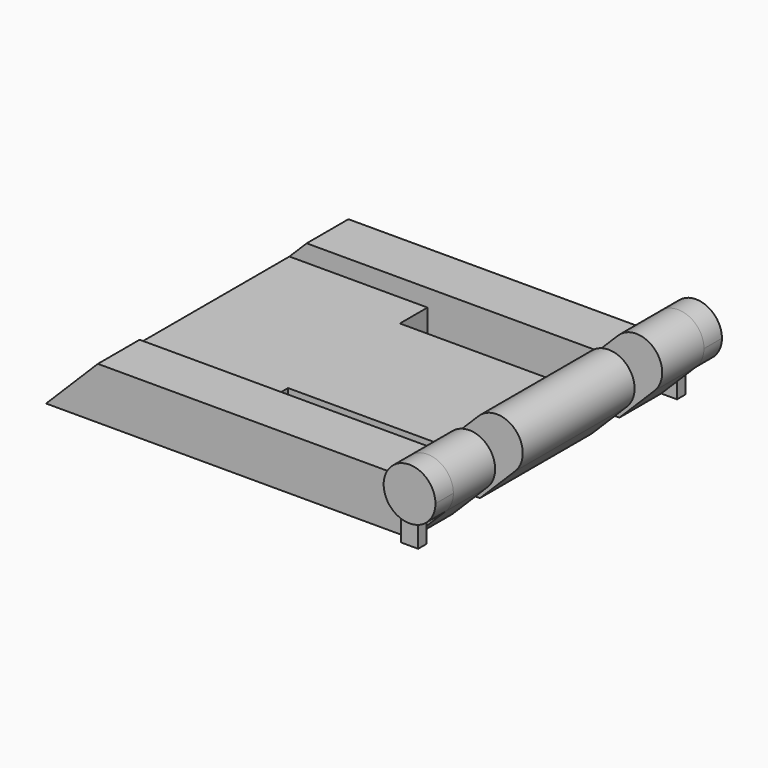
from build123d import *

# Parameters (mm, degrees)
F1_DEPTH  = 9.075
F3_DEPTH  = 1.3
F6_DEPTH  = 6.05
F7_W      = 15
F7_H      = 2
F8_DEPTH  = 4.601
F9_W      = 1
F9_H      = 0.6
F10_DEPTH = 3


with BuildPart() as f1:
    # F0 (on Front) → F1 (new body, symmetric)
    with BuildSketch(Plane.XZ):
        with BuildLine():
            Line((-3.0842823463, 3), (-6.0842823463, 0))
            Line((-6.0842823463, 0), (15.0370379973, 0))
            Line((15.0370379973, 0), (17.0763778255, 2.0393398282))
            ThreePointArc((17.0763778255, 2.0393398282), (17.0763778255, 4.1606601718), (14.9550574819, 4.1606601718))
            Line((14.9550574819, 4.1606601718), (13.7943973101, 3))
            Line((13.7943973101, 3), (-3.0842823463, 3))
        make_face()
    extrude(amount=F1_DEPTH, both=True)

    # F2 (on face) → F3 (join)
    with BuildSketch(Plane.XZ.offset(9.075)):
        with BuildLine():
            ThreePointArc((17.0763778255, 2.0393398282), (17.4015369525, 2.5259748515), (17.5157176537, 3.1))
            ThreePointArc((17.5157176537, 3.1), (16.5897428022, 4.4858192988), (14.9550574819, 4.1606601718))
            ThreePointArc((14.9550574819, 4.1606601718), (14.9550574819, 2.0393398282), (17.0763778255, 2.0393398282))
        make_face()
    extrude(amount=F3_DEPTH)

    # F4: F1 across plane


with BuildPart() as f1_1:
    add(f1.part)
    add(f1.part.mirror(Plane.XZ))

    # F5 (on Front) → F6 (cut, symmetric)
    with BuildSketch(Plane.XZ):
        Polygon((12.7943973101, 2), (13.7943973101, 3), (-3.0842823463, 3), (-4.0842823463, 2), align=None)
    extrude(amount=F6_DEPTH, both=True, mode=Mode.SUBTRACT)

    # F7 (on Top) → F8 (cut, through all)
    with BuildSketch(Plane.XY):
        with Locations((11.4157176537, -5.05)):
            Rectangle(F7_W, F7_H)
        with Locations((11.4157176537, 5.05)):
            Rectangle(F7_W, F7_H)
    extrude(amount=F8_DEPTH, mode=Mode.SUBTRACT)

    # F9 (on Top) → F10 (join)
    with BuildSketch(Plane.XY):
        with Locations((15.4550574819, 9.375)):
            Rectangle(F9_W, F9_H)
        with Locations((15.4550574819, -9.375)):
            Rectangle(F9_W, F9_H)
    extrude(amount=F10_DEPTH)


solid = f1_1.part
